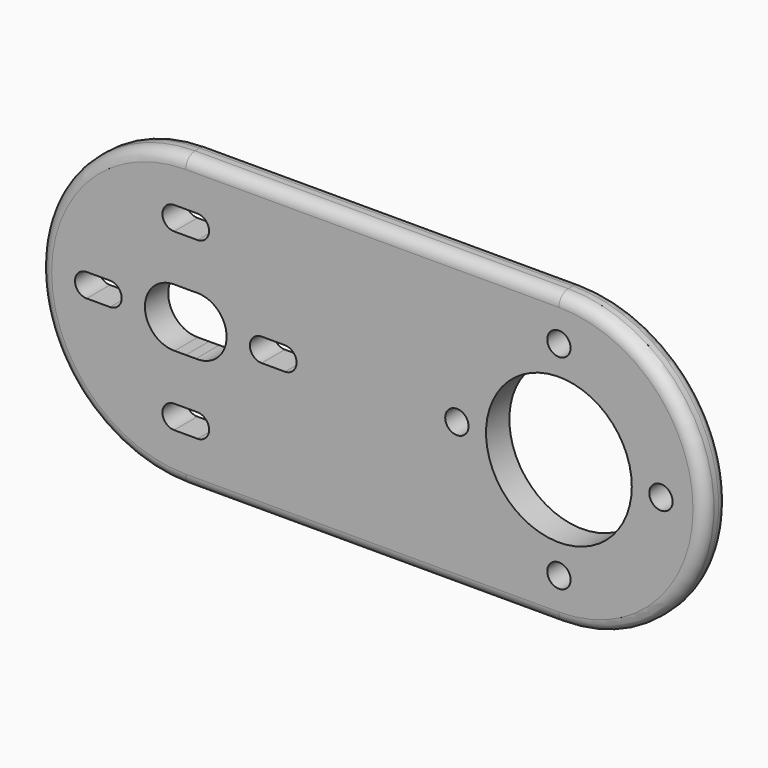
from build123d import *

# Parameters (mm, degrees)
F0_R     = 2
F0_R_2   = 12.5
F1_DEPTH = 5
F2_R     = 2


# Not quite as in the source:
# - two fillets or chamfers of one size are made in one step
# - ends of sketch curves that miss each other by under 0.0002 mm in the source are joined


with BuildPart() as f1:
    # F0 (on Front) → F1 (new body)
    with BuildSketch(Plane.XZ):
        with BuildLine():
            Line((30.4688991789, 25), (-33.5311008211, 25))
            ThreePointArc((-33.5311008211, 25), (-58.5311008211, 0), (-33.5311008211, -25))
            Line((-33.5311008211, -25), (30.4688991789, -25))
            ThreePointArc((30.4688991789, -25), (55.4688991789, 0), (30.4688991789, 25))
        make_face()
        with BuildLine():
            ThreePointArc((-31.5311008211, -13), (-29.5311008211, -15), (-31.5311008211, -17))
            Line((-31.5311008211, -17), (-35.5311008211, -17))
            ThreePointArc((-35.5311008211, -17), (-37.5311008211, -15), (-35.5311008211, -13))
            Line((-35.5311008211, -13), (-31.5311008211, -13))
        make_face(mode=Mode.SUBTRACT)
        with BuildLine():
            ThreePointArc((-35.6998849753, 5.0009525442), (-35.5197441178, 5.0037871123), (-35.3396179829, 5.0001348744))
            Line((-35.3396179829, 5.0001348744), (-33.7192871231, 4.9964573365))
            Line((-33.7192871231, 4.9964573365), (-31.8707135701, 4.9922617741))
            ThreePointArc((-31.8707135701, 4.9922617741), (-31.5197441178, 5.0037871123), (-31.1688305974, 4.9906687653))
            ThreePointArc((-31.1688305974, 4.9906687653), (-26.5369680234, -0.310889109), (-31.7905758861, -4.9970678533))
            Line((-31.7905758861, -4.9970678533), (-33.5226571845, -4.9999928705))
            ThreePointArc((-33.5226571845, -4.9999928705), (-33.5268790013, -4.9999982176), (-33.5311008211, -5))
            Line((-33.5311008211, -5), (-35.4576247605, -5.0032605078))
            ThreePointArc((-35.4576247605, -5.0032605078), (-40.5334343372, -0.1211356041), (-35.6998849753, 5.0009525442))
        make_face(mode=Mode.SUBTRACT)
        with Locations((30.4688991789, -17.5)):
            Circle(F0_R, mode=Mode.SUBTRACT)
        with BuildLine():
            ThreePointArc((-46.5311008211, 2), (-44.5311008211, 0), (-46.5311008211, -2))
            Line((-46.5311008211, -2), (-50.5311008211, -2))
            ThreePointArc((-50.5311008211, -2), (-52.5311008211, 0), (-50.5311008211, 2))
            Line((-50.5311008211, 2), (-46.5311008211, 2))
        make_face(mode=Mode.SUBTRACT)
        with BuildLine():
            ThreePointArc((-20.5311008211, -2), (-22.5311008211, 0), (-20.5311008211, 2))
            Line((-20.5311008211, 2), (-16.5311008211, 2))
            ThreePointArc((-16.5311008211, 2), (-14.5311008211, 0), (-16.5311008211, -2))
            Line((-16.5311008211, -2), (-20.5311008211, -2))
        make_face(mode=Mode.SUBTRACT)
        with BuildLine():
            ThreePointArc((-31.5311008211, 17), (-29.5311008211, 15), (-31.5311008211, 13))
            Line((-31.5311008211, 13), (-35.5311008211, 13))
            ThreePointArc((-35.5311008211, 13), (-37.5311008211, 15), (-35.5311008211, 17))
            Line((-35.5311008211, 17), (-31.5311008211, 17))
        make_face(mode=Mode.SUBTRACT)
        with Locations((12.9688991789, 0)):
            Circle(F0_R, mode=Mode.SUBTRACT)
        with Locations((30.4688991789, 0)):
            Circle(F0_R_2, mode=Mode.SUBTRACT)
        with Locations((47.9688991789, 0)):
            Circle(F0_R, mode=Mode.SUBTRACT)
        with Locations((30.4688991789, 17.5)):
            Circle(F0_R, mode=Mode.SUBTRACT)
    extrude(amount=-F1_DEPTH)

    # F2
    f2_edges = [f1.edges().sort_by_distance(p)[0] for p in [
        (55.468899, 5, 0),
        (-1.531101, 0, 25),
        (-1.531101, 5, 25),
        (-58.531101, 5, 0),
        (-1.531101, 5, -25),
        (-1.531101, 0, -25),
        (-58.531101, 0, 0),
        (55.468899, 0, 0),
    ]]
    fillet(f2_edges, radius=F2_R)


solid = f1.part
